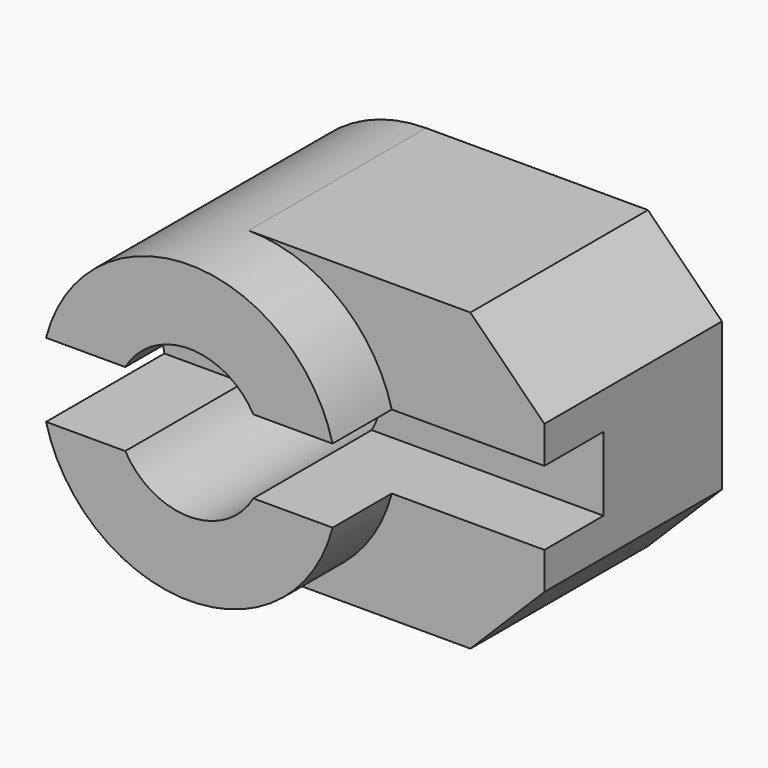
from build123d import *

# Parameters (mm, degrees)
F0_R     = 10
F0_R_2   = 5
F1_DEPTH = 20
F3_DEPTH = 15
F4_DEPTH = 15.001
F5_W     = 10
F5_H     = 5
F6_DEPTH = 30.001


with BuildPart() as f1:
    # F0 (on Front) → F1 (new body)
    with BuildSketch(Plane.XZ):
        Circle(F0_R)
        Circle(F0_R_2, mode=Mode.SUBTRACT)
    extrude(amount=F1_DEPTH)

    # F2 (on Front) → F3 (join)
    with BuildSketch(Plane.XZ):
        with BuildLine():
            Line((15, 10), (0, 10))
            ThreePointArc((0, 10), (7.0710678119, 7.0710678119), (10, 0))
            ThreePointArc((10, 0), (7.0710678119, -7.0710678119), (0, -10))
            Line((0, -10), (15, -10))
            Line((15, -10), (20, -5))
            Line((20, -5), (20, 5))
            Line((20, 5), (15, 10))
        make_face()
        with BuildLine():
            ThreePointArc((10, 0), (7.0710678119, 7.0710678119), (0, 10))
            ThreePointArc((0, 10), (-10, 0), (0, -10))
            ThreePointArc((0, -10), (7.0710678119, -7.0710678119), (10, 0))
        make_face()
    extrude(amount=F3_DEPTH)

    # F4 (cut, through all): a face of the model
    f4_faces = [f1.faces().sort_by_distance(p)[0] for p in [
        (0, -15, 0),
    ]]
    extrude(f4_faces, amount=-F4_DEPTH, mode=Mode.SUBTRACT)

    # F5 (on face) → F6 (cut, through all)
    with BuildSketch(Plane.YZ.offset(20)):
        with Locations((-15, 0)):
            Rectangle(F5_W, F5_H)
    extrude(amount=-F6_DEPTH, mode=Mode.SUBTRACT)


solid = f1.part
